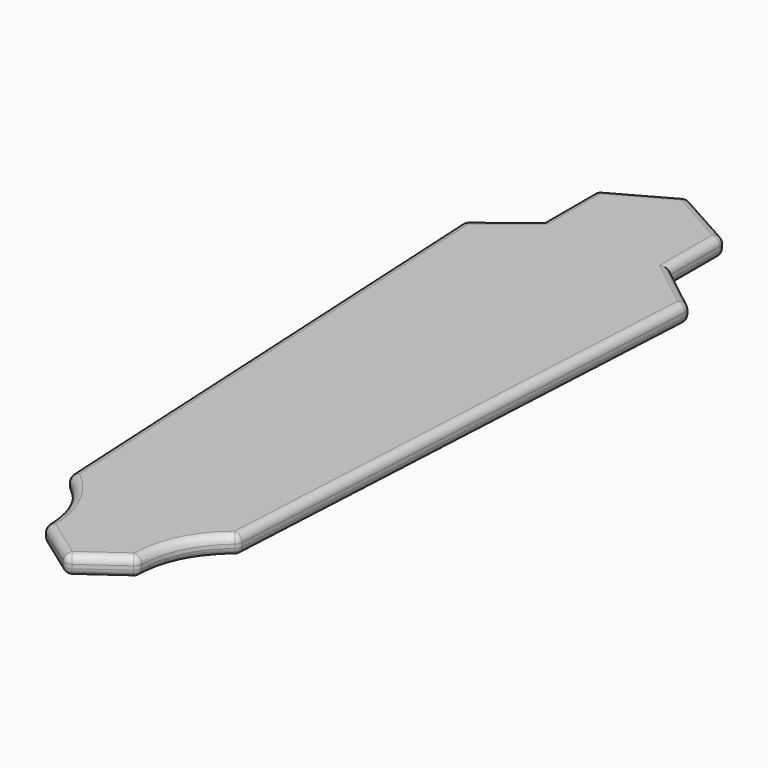
from build123d import *

# Parameters (mm, degrees)
F1_DEPTH = 12.7
F4_R     = 5.08


# Not quite as in the source:
# - a feature of the source that left no trace in its solid (it failed there, or was rolled back) is left out


with BuildPart() as f1:
    # F0 (on Top) → F1 (new body)
    with BuildSketch(Plane.XY):
        with BuildLine():
            Line((-44.0331279794, 186.6005068212), (-76.9840011597, 160.7028610468))
            Line((-76.9840011597, 160.7028610468), (-58.4838322918, -194.4155751852))
            add(Edge.make_bspline(
                [(-58.4838322918, -194.4155751852), (-46.5574619293, -203.8708319702), (-32.9955126884, -219.6695432067), (-32.7912761313, -246.9500899315)],
                knots=[0, 0, 0, 0, 58.4806180002, 58.4806180002, 58.4806180002, 58.4806180002], degree=3))
            Line((-32.7912761313, -246.9500899315), (-1.3338322918, -269.5246338844))
            Line((-1.3338322918, -269.5246338844), (30.1236115478, -246.9500899315))
            add(Edge.make_bspline(
                [(55.8161677082, -194.4155751852), (43.8897973458, -203.8708319702), (30.3278481049, -219.6695432067), (30.1236115478, -246.9500899315)],
                knots=[0, 0, 0, 0, 58.4806180002, 58.4806180002, 58.4806180002, 58.4806180002], degree=3))
            Line((55.8161677082, -194.4155751852), (74.3163365761, 160.7028610468))
            Line((74.3163365761, 160.7028610468), (41.3654633958, 186.6005068212))
            Line((41.3654633958, 186.6005068212), (41.3654633958, 231.4658612013))
            Line((41.3654633958, 231.4658612013), (-1.3338322918, 255.2684353284))
            Line((-1.3338322918, 255.2684353284), (-44.0331279794, 231.4658612013))
            Line((-44.0331279794, 231.4658612013), (-44.0331279794, 186.6005068212))
        make_face()
    extrude(amount=F1_DEPTH)

    # F4
    f4_edges = [f1.edges().sort_by_distance(p)[0] for p in [
        (-1.333832, 255.268435, 6.35),
        (41.365463, 231.465861, 6.35),
        (74.316337, 160.702861, 6.35),
        (-44.033128, 231.465861, 6.35),
        (-76.984001, 160.702861, 6.35),
        (-58.483832, -194.415575, 6.35),
        (-32.791276, -246.95009, 6.35),
        (-1.333832, -269.524634, 6.35),
        (30.123612, -246.95009, 6.35),
        (55.816168, -194.415575, 6.35),
        (-60.508565, 173.651684, 0),
        (-60.508565, 173.651684, 12.7),
        (-67.733917, -16.856357, 0),
        (-67.733917, -16.856357, 12.7),
        (-41.241754, -213.998349, 0),
        (-41.241754, -213.998349, 12.7),
        (-17.062554, -258.237362, 0),
        (-17.062554, -258.237362, 12.7),
        (14.39489, -258.237362, 0),
        (14.39489, -258.237362, 12.7),
        (38.574089, -213.998349, 0),
        (38.574089, -213.998349, 12.7),
        (65.066252, -16.856357, 0),
        (65.066252, -16.856357, 12.7),
        (57.8409, 173.651684, 0),
        (57.8409, 173.651684, 12.7),
        (41.365463, 209.033184, 0),
        (41.365463, 209.033184, 12.7),
        (20.015816, 243.367148, 0),
        (20.015816, 243.367148, 12.7),
        (-22.68348, 243.367148, 0),
        (-22.68348, 243.367148, 12.7),
        (-44.033128, 209.033184, 0),
        (-44.033128, 209.033184, 12.7),
    ]]
    fillet(f4_edges, radius=F4_R)


solid = f1.part
